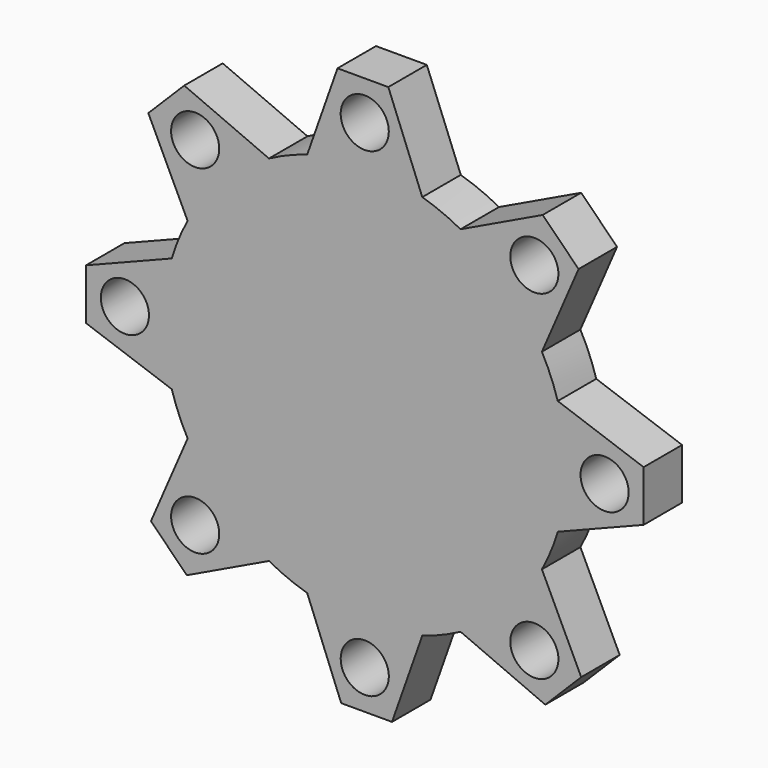
from build123d import *

# Parameters (mm, degrees)
F0_R            = 38.1
F1_DEPTH        = 6.35
F2_R            = 3.175
F3_DEPTH        = 6.351
F3_COPIES_COUNT = 8
F5_DEPTH        = 25.4


# Not quite as in the source:
# - a pattern or mirror of a feature is missing from the dataset's text; its kind, count and spacing are read off the source's solid


with BuildPart() as f1:
    # F0 (on Front) → F1 (new body)
    with BuildSketch(Plane.XZ):
        Circle(F0_R)
    extrude(amount=F1_DEPTH)

    # F2 (on face) → F3 (cut, through all)
    with BuildSketch(Plane.XZ.offset(6.35)):
        with Locations((0, 31.6533222795)):
            Circle(F2_R)
    f3 = extrude(amount=-F3_DEPTH, mode=Mode.SUBTRACT)

    # F3_copies: F3 ×8 about axis
    f3_copies_axis = Axis((0, 0, 0), (0, 1, 0))
    for i in range(1, F3_COPIES_COUNT):
        add(f3.rotate(f3_copies_axis, i * 360 / F3_COPIES_COUNT), mode=Mode.SUBTRACT)

    # F4 (on Front) → F5 (intersect)
    with BuildSketch(Plane.XZ):
        with BuildLine():
            Line((3.1097339764, 36.7998792025), (-3.5963490721, 36.7998792025))
            Line((-3.5963490721, 36.7998792025), (-7.5950432294, 25.4702454258))
            ThreePointArc((-7.5950432294, 25.4702454258), (-10.1728112394, 24.5546735917), (-12.6428176097, 23.378991565))
            Line((-12.6428176097, 23.378991565), (-23.8225301486, 28.2203581134))
            Line((-23.8225301486, 28.2203581134), (-28.5644469474, 23.4784413146))
            Line((-28.5644469474, 23.4784413146), (-23.38068983, 12.6396766882))
            ThreePointArc((-23.38068983, 12.6396766882), (-24.5560400177, 10.1695123954), (-25.4712655381, 7.5916214078))
            Line((-25.4712655381, 7.5916214078), (-36.7998792025, 3.1097339764))
            Line((-36.7998792025, 3.1097339764), (-36.7998792025, -3.5963490721))
            Line((-36.7998792025, -3.5963490721), (-25.4702454258, -7.5950432294))
            ThreePointArc((-25.4702454258, -7.5950432294), (-24.5546735917, -10.1728112394), (-23.378991565, -12.6428176097))
            Line((-23.378991565, -12.6428176097), (-28.2203581134, -23.8225301486))
            Line((-28.2203581134, -23.8225301486), (-23.4784413146, -28.5644469474))
            Line((-23.4784413146, -28.5644469474), (-12.6396766882, -23.38068983))
            ThreePointArc((-12.6396766882, -23.38068983), (-10.1695123954, -24.5560400177), (-7.5916214078, -25.4712655381))
            Line((-7.5916214078, -25.4712655381), (-3.1097339764, -36.7998792025))
            Line((-3.1097339764, -36.7998792025), (3.5963490721, -36.7998792025))
            Line((3.5963490721, -36.7998792025), (7.5950432294, -25.4702454258))
            ThreePointArc((7.5950432294, -25.4702454258), (10.1728112394, -24.5546735917), (12.6428176097, -23.378991565))
            Line((12.6428176097, -23.378991565), (23.8225301486, -28.2203581134))
            Line((23.8225301486, -28.2203581134), (28.5644469474, -23.4784413146))
            Line((28.5644469474, -23.4784413146), (23.38068983, -12.6396766882))
            ThreePointArc((23.38068983, -12.6396766882), (24.5560400177, -10.1695123954), (25.4712655381, -7.5916214078))
            Line((25.4712655381, -7.5916214078), (36.7998792025, -3.1097339764))
            Line((36.7998792025, -3.1097339764), (36.7998792025, 3.5963490721))
            Line((36.7998792025, 3.5963490721), (25.4702454258, 7.5950432294))
            ThreePointArc((25.4702454258, 7.5950432294), (24.5546735917, 10.1728112394), (23.378991565, 12.6428176097))
            Line((23.378991565, 12.6428176097), (28.2203581134, 23.8225301486))
            Line((28.2203581134, 23.8225301486), (23.4784413146, 28.5644469474))
            Line((23.4784413146, 28.5644469474), (12.6396766882, 23.38068983))
            ThreePointArc((12.6396766882, 23.38068983), (10.1695123954, 24.5560400177), (7.5916214078, 25.4712655381))
            Line((7.5916214078, 25.4712655381), (3.1097339764, 36.7998792025))
        make_face()
    extrude(amount=F5_DEPTH, mode=Mode.INTERSECT)


solid = f1.part
